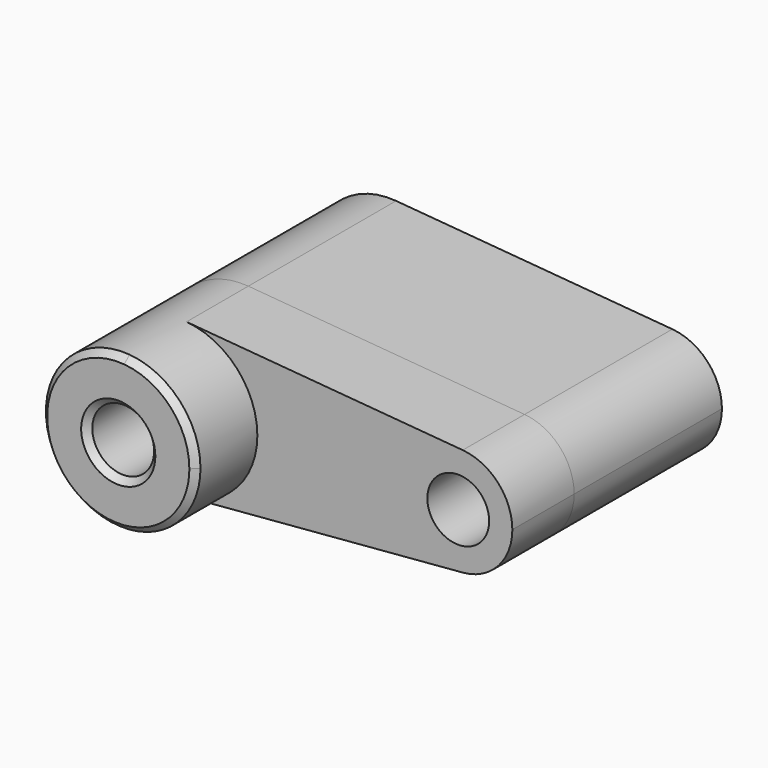
from build123d import *

# Parameters (mm, degrees)
F0_R          = 10
F1_DEPTH      = 25
F2_DEPTH      = 50
F3_SIZE       = 2
F5_DEPTH      = 25
F5_DEPTH_BACK = 59.7565770149


# Not quite as in the source:
# - the program builds the solid bodies; features that only make, move or delete a surface that nothing else refers to are left out


with BuildPart() as f1:
    # F0 (on Front) → F1 (new body)
    with BuildSketch(Plane.XZ):
        with BuildLine():
            ThreePointArc((2.0833333333, -24.9130432148), (18.3995018048, -16.9250800097), (25, 0))
            ThreePointArc((25, 0), (18.3995018048, 16.9250800097), (2.0833333333, 24.9130432148))
            ThreePointArc((2.0833333333, 24.9130432148), (-25, 0), (2.0833333333, -24.9130432148))
        make_face()
        Circle(F0_R, mode=Mode.SUBTRACT)
        with BuildLine():
            ThreePointArc((2.0833333333, 24.9130432148), (18.3995018048, 16.9250800097), (25, 0))
            ThreePointArc((25, 0), (18.3995018048, -16.9250800097), (2.0833333333, -24.9130432148))
            Line((2.0833333333, -24.9130432148), (91.4583333333, -17.4391302504))
            ThreePointArc((91.4583333333, -17.4391302504), (72.5, 0), (91.4583333333, 17.4391302504))
            Line((91.4583333333, 17.4391302504), (2.0833333333, 24.9130432148))
        make_face()
        with BuildLine():
            ThreePointArc((107.5, 0), (102.8796512634, 11.8475560068), (91.4583333333, 17.4391302504))
            ThreePointArc((91.4583333333, 17.4391302504), (72.5, 0), (91.4583333333, -17.4391302504))
            ThreePointArc((91.4583333333, -17.4391302504), (102.8796512634, -11.8475560068), (107.5, 0))
        make_face()
        with Locations((90, 0)):
            Circle(F0_R, mode=Mode.SUBTRACT)
    extrude(amount=F1_DEPTH)

    # F0 (on Front) → F2 (join)
    with BuildSketch(Plane.XZ):
        with BuildLine():
            ThreePointArc((2.0833333333, -24.9130432148), (18.3995018048, -16.9250800097), (25, 0))
            ThreePointArc((25, 0), (18.3995018048, 16.9250800097), (2.0833333333, 24.9130432148))
            ThreePointArc((2.0833333333, 24.9130432148), (-25, 0), (2.0833333333, -24.9130432148))
        make_face()
        Circle(F0_R, mode=Mode.SUBTRACT)
    extrude(amount=F2_DEPTH)

    # F3
    f3_edges = [f1.edges().sort_by_distance(p)[0] for p in [
        (-2.083333, -50, 24.913043),
        (-10, -50, 0),
        (80, -25, 0),
    ]]
    chamfer(f3_edges, length=F3_SIZE)

    # F0 (on Front) → F5 (join, two sides)
    with BuildSketch(Plane.XZ) as f5_sk:
        with BuildLine():
            ThreePointArc((2.0833333333, -24.9130432148), (18.3995018048, -16.9250800097), (25, 0))
            ThreePointArc((25, 0), (18.3995018048, 16.9250800097), (2.0833333333, 24.9130432148))
            ThreePointArc((2.0833333333, 24.9130432148), (-25, 0), (2.0833333333, -24.9130432148))
        make_face()
        Circle(F0_R, mode=Mode.SUBTRACT)
        with BuildLine():
            ThreePointArc((2.0833333333, 24.9130432148), (18.3995018048, 16.9250800097), (25, 0))
            ThreePointArc((25, 0), (18.3995018048, -16.9250800097), (2.0833333333, -24.9130432148))
            Line((2.0833333333, -24.9130432148), (91.4583333333, -17.4391302504))
            ThreePointArc((91.4583333333, -17.4391302504), (72.5, 0), (91.4583333333, 17.4391302504))
            Line((91.4583333333, 17.4391302504), (2.0833333333, 24.9130432148))
        make_face()
        with BuildLine():
            ThreePointArc((107.5, 0), (102.8796512634, 11.8475560068), (91.4583333333, 17.4391302504))
            ThreePointArc((91.4583333333, 17.4391302504), (72.5, 0), (91.4583333333, -17.4391302504))
            ThreePointArc((91.4583333333, -17.4391302504), (102.8796512634, -11.8475560068), (107.5, 0))
        make_face()
        with Locations((90, 0)):
            Circle(F0_R, mode=Mode.SUBTRACT)
    extrude(amount=F5_DEPTH)
    extrude(f5_sk.sketch, amount=-F5_DEPTH_BACK)


solid = f1.part
